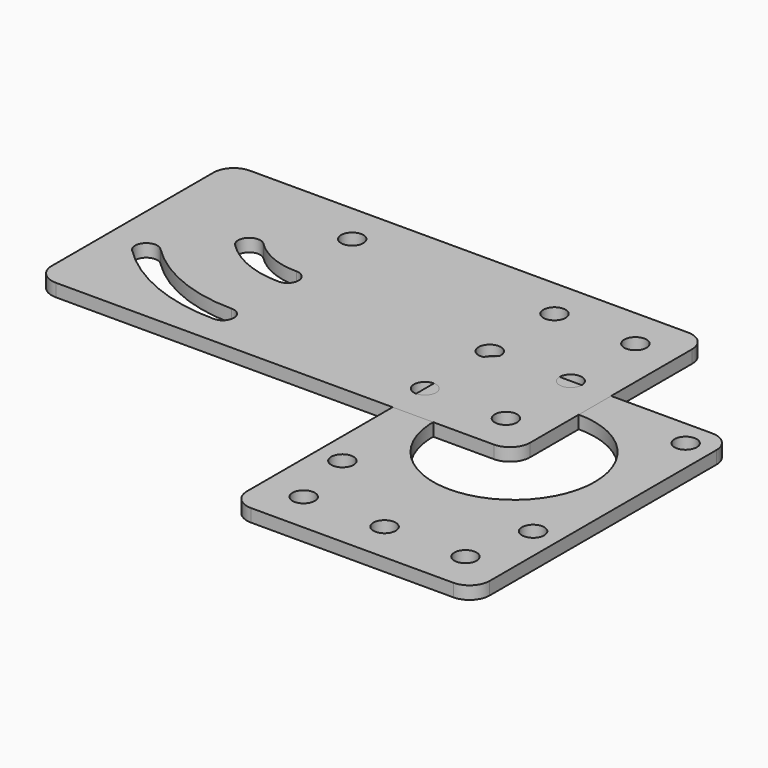
from build123d import *

# Parameters (mm, degrees)
F0_R     = 2.75
F0_R_2   = 20
F1_DEPTH = 3.175
F2_R     = 2.75
F3_DEPTH = 3.175


# Not quite as in the source:
# - a length typed as a fraction of an inch, garbled in the dataset ("3 / 203.2 mm" for 3/8 in), is restored


with BuildPart() as f1:
    # F0 (on Top) → F1 (new body)
    with BuildSketch(Plane.XY):
        with BuildLine():
            Line((30, -45), (30, -30))
            Line((30, -30), (30, 25))
            ThreePointArc((30, 25), (28.5355339059, 28.5355339059), (25, 30))
            Line((25, 30), (-25, 30))
            ThreePointArc((-25, 30), (-28.5355339059, 28.5355339059), (-30, 25))
            Line((-30, 25), (-30, -30))
            Line((-30, -30), (-30, -45))
            ThreePointArc((-30, -45), (-28.5355339059, -48.5355339059), (-25, -50))
            Line((-25, -50), (25, -50))
            ThreePointArc((25, -50), (28.5355339059, -48.5355339059), (30, -45))
        make_face()
        with Locations((-20, -40)):
            Circle(F0_R, mode=Mode.SUBTRACT)
        with Locations((0, -40)):
            Circle(F0_R, mode=Mode.SUBTRACT)
        with Locations((-23.57, -23.57)):
            Circle(F0_R, mode=Mode.SUBTRACT)
        with Locations((20, -40)):
            Circle(F0_R, mode=Mode.SUBTRACT)
        with Locations((23.57, -23.57)):
            Circle(F0_R, mode=Mode.SUBTRACT)
        Circle(F0_R_2, mode=Mode.SUBTRACT)
        with Locations((-23.57, 23.57)):
            Circle(F0_R, mode=Mode.SUBTRACT)
        with Locations((23.57, 23.57)):
            Circle(F0_R, mode=Mode.SUBTRACT)
    extrude(amount=F1_DEPTH)


with BuildPart() as f3:
    # F2 (on Top) → F3 (new body)
    with BuildSketch(Plane.XY):
        with BuildLine():
            Line((-113.2842712475, 0), (-5, 0))
            ThreePointArc((-5, 0), (-1.4644660941, 1.4644660941), (0, 5))
            Line((0, 5), (0, 55))
            ThreePointArc((0, 55), (-1.4644660941, 58.5355339059), (-5, 60))
            Line((-5, 60), (-113.2842712475, 60))
            ThreePointArc((-113.2842712475, 60), (-116.8198051534, 58.5355339059), (-118.2842712475, 55))
            Line((-118.2842712475, 55), (-118.2842712475, 5))
            ThreePointArc((-118.2842712475, 5), (-116.8198051534, 1.4644660941), (-113.2842712475, 0))
        make_face()
        with BuildLine():
            ThreePointArc((-110.2288148957, 19.7711851043), (-110.2288148957, 23.6602724008), (-106.3397275992, 23.6602724008))
            ThreePointArc((-106.3397275992, 23.6602724008), (-94.2549578556, 15.585487414), (-80, 12.75))
            ThreePointArc((-80, 12.75), (-77.25, 10), (-80, 7.25))
            ThreePointArc((-80, 7.25), (-96.3597167336, 10.5041499851), (-110.2288148957, 19.7711851043))
        make_face(mode=Mode.SUBTRACT)
        with Locations((-30, 10)):
            Circle(F2_R, mode=Mode.SUBTRACT)
        with Locations((-10, 10)):
            Circle(F2_R, mode=Mode.SUBTRACT)
        with BuildLine():
            ThreePointArc((-96.086679272, 33.913320728), (-96.086679272, 37.8024080245), (-92.1975919755, 37.8024080245))
            ThreePointArc((-92.1975919755, 37.8024080245), (-86.6012892083, 34.0630780642), (-80, 32.75))
            ThreePointArc((-80, 32.75), (-77.25, 30), (-80, 27.25))
            ThreePointArc((-80, 27.25), (-88.7060480863, 28.9817406354), (-96.086679272, 33.913320728))
        make_face(mode=Mode.SUBTRACT)
        with Locations((-80, 50)):
            Circle(F2_R, mode=Mode.SUBTRACT)
        with Locations((-30, 30)):
            Circle(F2_R, mode=Mode.SUBTRACT)
        with Locations((-10, 30)):
            Circle(F2_R, mode=Mode.SUBTRACT)
        with Locations((-30, 50)):
            Circle(F2_R, mode=Mode.SUBTRACT)
        with Locations((-10, 50)):
            Circle(F2_R, mode=Mode.SUBTRACT)
    extrude(amount=F3_DEPTH)


solid = Compound([f1.part, f3.part])
